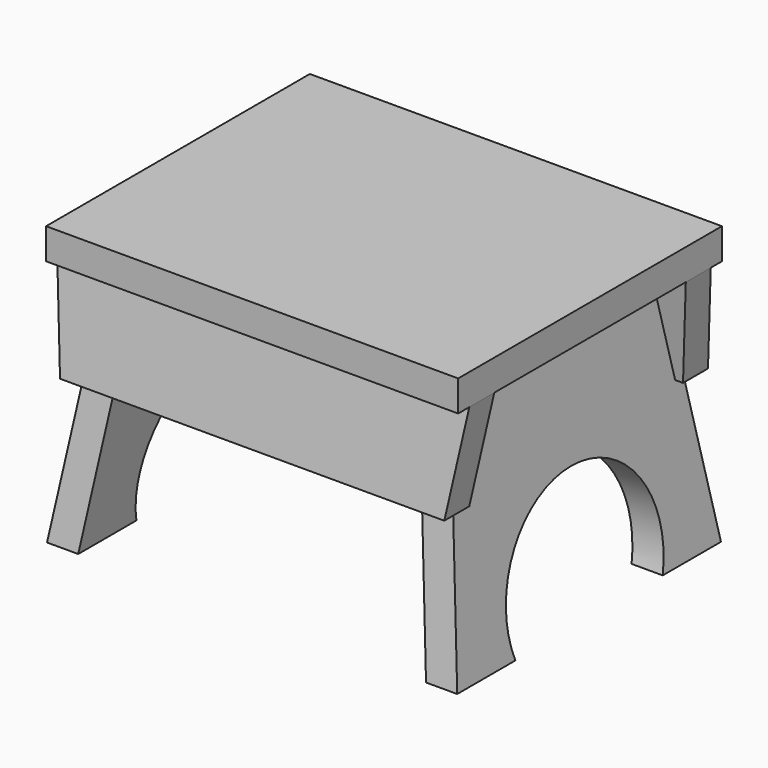
from build123d import *

# Parameters (mm, degrees)
F1_DEPTH       = 101.6
F2_DEPTH       = 101.6
F2_DEPTH_BACK  = 101.6
F4_DEPTH       = 127.001
F4_DEPTH_BACK  = 127.001
F6_DEPTH       = 127
F9_DEPTH       = 127.001
F9_DEPTH_BACK  = 127.001
F10_DEPTH      = 101.6010000004
F10_DEPTH_BACK = 101.6010000004


# Not quite as in the source:
# - a feature names something its author has since deleted; it is built from what else it names


with BuildPart() as f1:
    # F0 (on Front) → F1 (new body, symmetric)
    with BuildSketch(Plane.XZ):
        Polygon((127, -9.525), (127, 9.525), (-127, 9.525), (-127, -9.525), (-104.9997227219, -9.525), (-85.7625074654, -9.525), (0, -9.525), (85.7625074654, -9.525), (104.9997227219, -9.525), align=None)
    extrude(amount=F1_DEPTH, both=True)


with BuildPart() as f2:
    # F0 (on Front) → F2 (new body, two sides)
    with BuildSketch(Plane.XZ) as f2_sk:
        Polygon((-94.3297724402, -70.4842578052), (-113.5669876967, -70.4842578052), (-126.4181459306, -161.925), (-107.1809306741, -161.925), align=None)
        Polygon((-85.7625074654, -9.525), (-104.9997227219, -9.525), (-113.5669876967, -70.4842578052), (-94.3297724402, -70.4842578052), align=None)
    extrude(amount=F2_DEPTH)
    extrude(f2_sk.sketch, amount=-F2_DEPTH_BACK)


with BuildPart() as f2b:
    # F0 (on Front) → F2, piece 2 (new body, two sides)
    with BuildSketch(Plane.XZ) as f2_2_sk:
        Polygon((113.5669876967, -70.4842578052), (104.9997227219, -9.525), (85.7625074654, -9.525), (94.3297724402, -70.4842578052), align=None)
        Polygon((126.4181459306, -161.925), (113.5669876967, -70.4842578052), (94.3297724402, -70.4842578052), (107.1809306741, -161.925), align=None)
    extrude(amount=F2_DEPTH)
    extrude(f2_2_sk.sketch, amount=-F2_DEPTH_BACK)


with BuildPart() as f4_tool:
    # F3 (on Right) → F4 (new body, two sides)
    with BuildSketch(Plane.YZ) as f4_sk:
        Polygon((-101.6000000004, -161.925), (-80.1815767917, -9.525), (-101.6000000004, -9.525), align=None)
        Polygon((101.5999999998, -161.925), (101.5999999997, -9.525), (80.1815767917, -9.525), align=None)
    extrude(amount=-F4_DEPTH)
    extrude(f4_sk.sketch, amount=F4_DEPTH_BACK)


with BuildPart() as f2_1:
    add(f2.part)

    # F4: cut by f4_tool
    add(f4_tool.part, mode=Mode.SUBTRACT)


with BuildPart() as f2b_1:
    add(f2b.part)

    # F4: cut by f4_tool
    add(f4_tool.part, mode=Mode.SUBTRACT)


with BuildPart() as f6:
    # F5 (on Right) → F6 (new body, symmetric)
    with BuildSketch(Plane.YZ):
        Polygon((80.1815767913, -9.525), (73.7691717062, -9.525), (82.336436681, -70.4842578052), (101.5736519375, -70.4842578052), (93.0063869627, -9.525), align=None)
    extrude(amount=F6_DEPTH, both=True)

    # F7: cut F2
    add(f2_1.part, mode=Mode.SUBTRACT)

    # F8: cut F2b
    add(f2b_1.part, mode=Mode.SUBTRACT)


with BuildPart() as f6b:
    # F5 (on Right) → F6, piece 2 (new body, symmetric)
    with BuildSketch(Plane.YZ):
        Polygon((-101.5736519375, -70.4842578052), (-82.336436681, -70.4842578052), (-73.7691717062, -9.525), (-80.1815767915, -9.525), (-93.0063869627, -9.525), align=None)
    extrude(amount=F6_DEPTH, both=True)

    # F7: cut F2
    add(f2_1.part, mode=Mode.SUBTRACT)

    # F8: cut F2b
    add(f2b_1.part, mode=Mode.SUBTRACT)


with BuildPart() as f9_tool:
    # F3 (on Right) → F9 (new body, two sides)
    with BuildSketch(Plane.YZ) as f9_sk:
        with BuildLine():
            Line((-56.7326918244, -161.925), (56.7326918244, -161.925))
            ThreePointArc((56.7326918244, -161.925), (0, -83.0369391017), (-56.7326918244, -161.925))
        make_face()
    extrude(amount=-F9_DEPTH)
    extrude(f9_sk.sketch, amount=F9_DEPTH_BACK)


with BuildPart() as f2_2:
    add(f2_1.part)

    # F9: cut by f9_tool
    add(f9_tool.part, mode=Mode.SUBTRACT)


with BuildPart() as f2b_2:
    add(f2b_1.part)

    # F9: cut by f9_tool
    add(f9_tool.part, mode=Mode.SUBTRACT)


with BuildPart() as f10_tool:
    # F0 (on Front) → F10 (new body, two sides)
    with BuildSketch(Plane.XZ) as f10_sk:
        Polygon((127, -70.4842578052), (127, -9.525), (118.4327350252, -70.4842578052), align=None)
        Polygon((-118.4327350252, -70.4842578052), (-127, -9.525), (-127, -70.4842578052), align=None)
    extrude(amount=F10_DEPTH)
    extrude(f10_sk.sketch, amount=-F10_DEPTH_BACK)


with BuildPart() as f6_1:
    add(f6.part)

    # F10: cut by f10_tool
    add(f10_tool.part, mode=Mode.SUBTRACT)


with BuildPart() as f6b_1:
    add(f6b.part)

    # F10: cut by f10_tool
    add(f10_tool.part, mode=Mode.SUBTRACT)


solid = Compound([f1.part, f2_2.part, f2b_2.part, f6_1.part, f6b_1.part])
